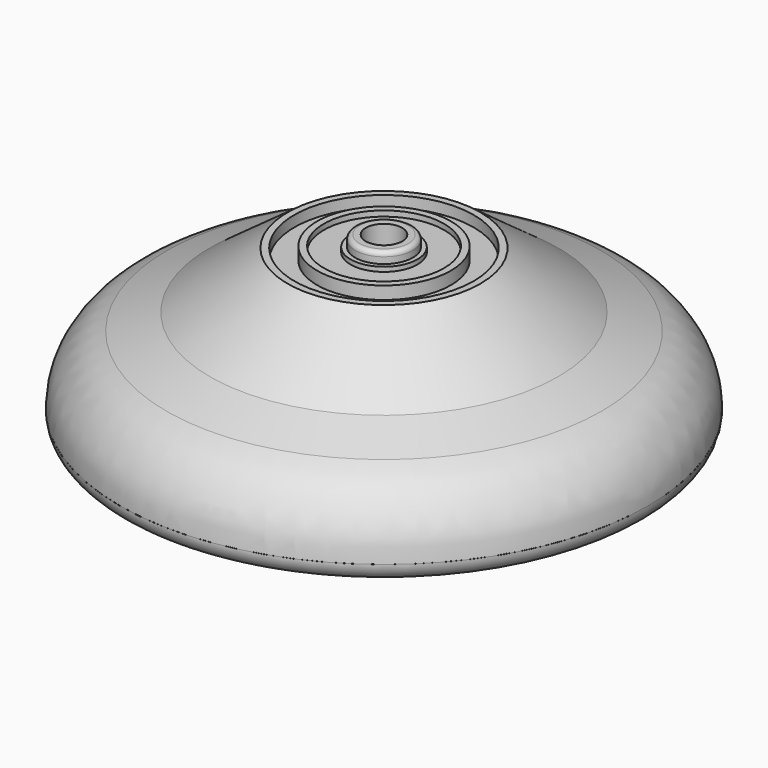
from build123d import *

# Parameters (mm, degrees)
F2_R     = 25
F3_R     = 8
F4_R     = 0.5
F5_R     = 2
F8_DEPTH = 3.5


# Not quite as in the source:
# - a feature names something its author has since deleted; it is built from what else it names


with BuildPart() as f1:
    # F0 (on Front) → F1 (revolve)
    with BuildSketch(Plane.XZ):
        Polygon((3.175, -1.2), (2, -1.2), (2, -9), (12.8490433491, -10.9498299199), (19.1417375121, -20), (29, -20), (29, -12.5), (19.1417375121, -8.7112029778), (10.6, -2.5), (9.85, -2.5), (9.85, -3.7), (7.35, -3.7), (7.35, -2.3), (6.6, -2.3), (6.6, -2.9), (3.675, -2.9), (3.675, -2.4), (3.175, -2.4), align=None)
    revolve(axis=Axis((0, 0, -7.3547498323), (0, 0, -1)))

    # F2
    f2_edges = [f1.edges().sort_by_distance(p)[0] for p in [
        (-12.849043, 0, -10.94983),
    ]]
    fillet(f2_edges, radius=F2_R)

    # F3
    f3_edges = [f1.edges().sort_by_distance(p)[0] for p in [
        (-29, 0, -12.5),
    ]]
    fillet(f3_edges, radius=F3_R)

    # F4
    f4_edges = [f1.edges().sort_by_distance(p)[0] for p in [
        (-3.175, 0, -1.2),
    ]]
    fillet(f4_edges, radius=F4_R)

    # F5
    f5_edges = [f1.edges().sort_by_distance(p)[0] for p in [
        (-29, 0, -20),
        (-19.141738, 0, -20),
    ]]
    fillet(f5_edges, radius=F5_R)

    # F7 (on offset) → F8 (cut)
    with BuildSketch(Plane.XY.offset(-6.5)):
        Polygon((2.0207259422, -3.5), (4.0414518843, 0), (2.0207259422, 3.5), (-2.0207259422, 3.5), (-4.0414518843, 0), (-2.0207259422, -3.5), align=None)
    extrude(amount=-F8_DEPTH, mode=Mode.SUBTRACT)


solid = f1.part
